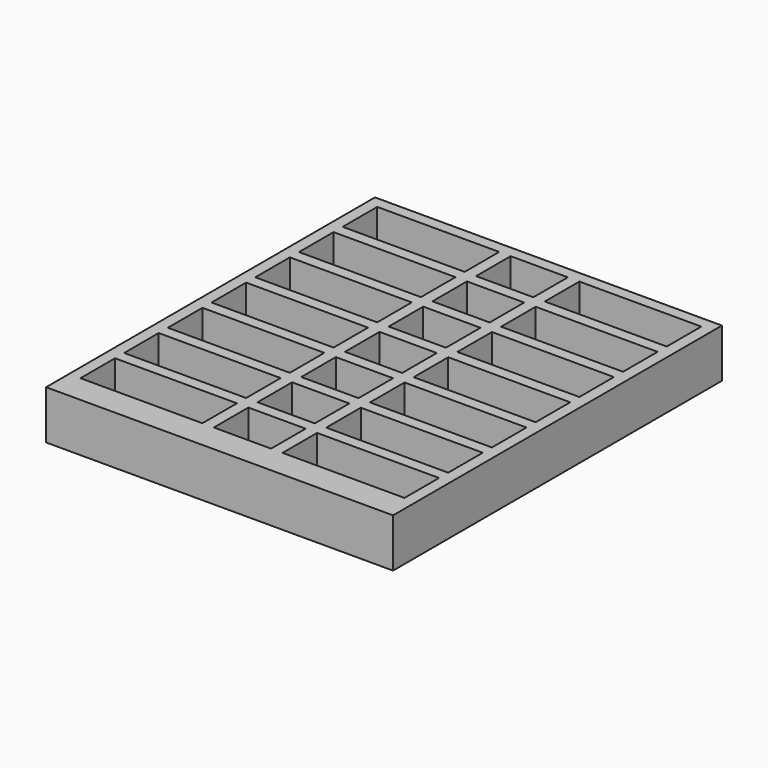
from build123d import *

# Parameters (mm, degrees)
F0_W     = 60.6
F0_H     = 71.8
F1_DEPTH = 8.5
F2_W     = 56.6
F2_H     = 64.7999969125
F3_DEPTH = 6
F4_W     = 10
F4_H     = 7.5428567018
F5_DEPTH = 6


with BuildPart() as f1:
    # F0 (on Top) → F1 (new body)
    with BuildSketch(Plane.XY):
        with Locations((30.3, 35.9)):
            Rectangle(F0_W, F0_H)
    extrude(amount=F1_DEPTH)

    # F2 (on face) → F3 (cut)
    with BuildSketch(Plane.XY.offset(8.5)):
        with Locations((30.3, 37.3999984562)):
            Rectangle(F2_W, F2_H)
    extrude(amount=-F3_DEPTH, mode=Mode.SUBTRACT)

    # F4 (on face) → F5 (join)
    with BuildSketch(Plane.XY.offset(2.5)):
        Polygon((25.3, 69.7999969125), (23.3, 69.7999969125), (23.3, 62.2571402107), (2, 62.2571402107), (2, 60.2571402107), (23.3, 60.2571402107), (23.3, 52.7142835089), (2, 52.7142835089), (2, 50.7142835089), (23.3, 50.7142835089), (23.3, 43.1714268071), (2, 43.1714268071), (2, 41.1714268071), (23.3, 41.1714268071), (23.3, 33.6285701053), (2, 33.6285701053), (2, 31.6285701053), (23.3, 31.6285701053), (23.3, 24.0857134036), (2, 24.0857134036), (2, 22.0857134036), (23.3, 22.0857134036), (23.3, 14.5428567018), (2, 14.5428567018), (2, 12.5428567018), (23.3, 12.5428567018), (23.3, 5), (25.3, 5), (25.3, 12.5428567018), (35.3, 12.5428567018), (35.3, 5), (37.3, 5), (37.3, 12.5428567018), (58.6, 12.5428567018), (58.6, 14.5428567018), (37.3, 14.5428567018), (37.3, 22.0857134036), (58.6, 22.0857134036), (58.6, 24.0857134036), (37.3, 24.0857134036), (37.3, 31.6285701053), (58.6, 31.6285701053), (58.6, 33.6285701053), (37.3, 33.6285701053), (37.3, 41.1714268071), (58.6, 41.1714268071), (58.6, 43.1714268071), (37.3, 43.1714268071), (37.3, 50.7142835089), (58.6, 50.7142835089), (58.6, 52.7142835089), (37.3, 52.7142835089), (37.3, 60.2571402107), (58.6, 60.2571402107), (58.6, 62.2571402107), (37.3, 62.2571402107), (37.3, 69.7999969125), (35.3, 69.7999969125), (35.3, 62.2571402107), (25.3, 62.2571402107), align=None)
        with Locations((30.3, 18.3142850527)):
            Rectangle(F4_W, F4_H, mode=Mode.SUBTRACT)
        with Locations((30.3, 27.8571417545)):
            Rectangle(F4_W, F4_H, mode=Mode.SUBTRACT)
        with Locations((30.3, 37.3999984562)):
            Rectangle(F4_W, F4_H, mode=Mode.SUBTRACT)
        with Locations((30.3, 46.942855158)):
            Rectangle(F4_W, F4_H, mode=Mode.SUBTRACT)
        with Locations((30.3, 56.4857118598)):
            Rectangle(F4_W, F4_H, mode=Mode.SUBTRACT)
    extrude(amount=F5_DEPTH)


with BuildPart() as f6_1:
    # F6: copy of F1
    add(f1.part)


solid = f1.part
